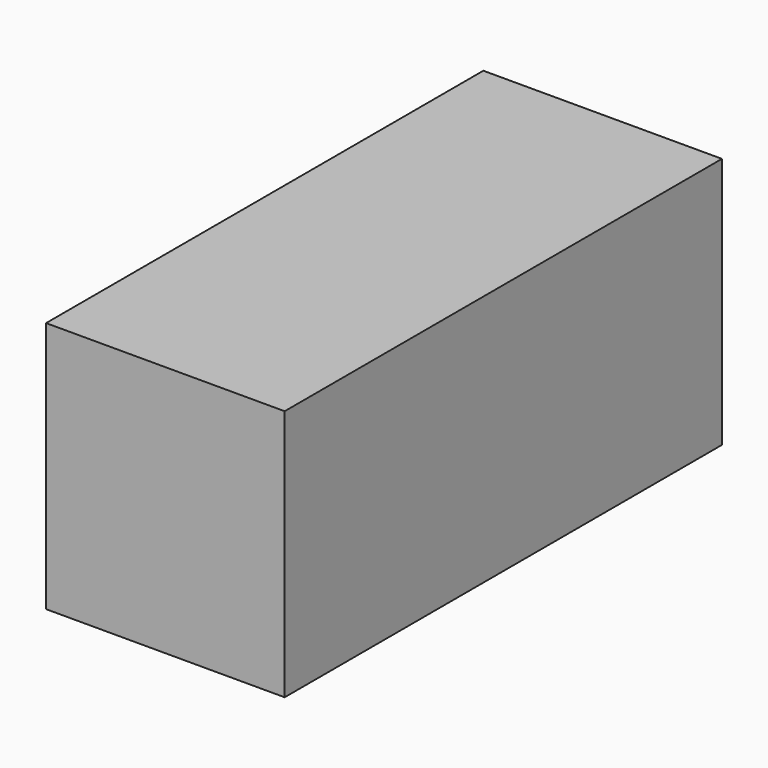
from build123d import *

# Parameters (mm, degrees)
F1_DEPTH = 99.314


# Not quite as in the source:
# - the program builds the solid bodies; features that only make, move or delete a surface that nothing else refers to are left out


with BuildPart() as f1:
    # F0 (on Front) → F1 (new body)
    with BuildSketch(Plane.XZ):
        Polygon((-70.2204668219, 30.4097067565), (-26.8668271601, 30.4097067565), (-26.8668271601, 76.1718861759), (-40.1111178976, 76.1718861759), (-70.2204668219, 76.1718861759), align=None)
    extrude(amount=F1_DEPTH)


solid = f1.part
